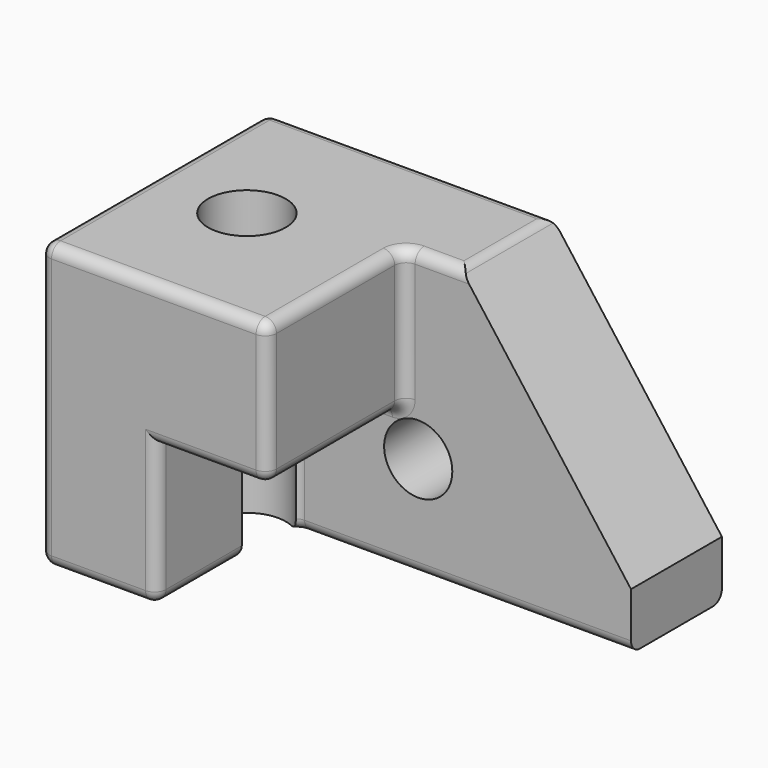
from build123d import *

# Parameters (mm, degrees)
F0_W     = 203.2
F0_H     = 127
F1_DEPTH = 127
F3_DEPTH = 76.2
F4_SIZE2 = 101.6
F4_SIZE  = 76.2
F5_R     = 5.08
F6_R     = 15.24
F7_DEPTH = 50.8
F8_R     = 17.3644725526
F9_DEPTH = 127


with BuildPart() as f1:
    # F0 (on Front) → F1 (new body)
    with BuildSketch(Plane.XZ):
        Rectangle(F0_W, F0_H)
    extrude(amount=F1_DEPTH)

    # F2 (on face) → F3 (cut)
    with BuildSketch(Plane.XZ.offset(127)):
        Polygon((101.6, 63.5), (0, 63.5), (0, 0), (-49.4145452976, 0), (-49.4145452976, -63.5), (101.6, -63.5), align=None)
    extrude(amount=-F3_DEPTH, mode=Mode.SUBTRACT)

    # F4
    f4_edges = [f1.edges().sort_by_distance(p)[0] for p in [
        (101.6, -25.4, 63.5),
    ]]
    f4_side = f1.faces().sort_by_distance((-21.771429, -52.614286, 63.5))[0]
    chamfer(f4_edges, length=F4_SIZE, length2=F4_SIZE2, reference=f4_side)

    # F5
    f5_edges = [f1.edges().sort_by_distance(p)[0] for p in [
        (25.4, -25.4, 63.5),
        (12.7, -50.8, 63.5),
        (0, -88.9, 63.5),
        (-50.8, -127, 63.5),
        (-101.6, -63.5, 63.5),
        (-38.1, 0, 63.5),
        (-101.6, -127, 0),
        (-49.414545, -127, -31.75),
        (-24.707273, -127, 0),
        (0, -88.9, 0),
        (0, -127, 31.75),
        (-75.507273, -127, -63.5),
        (0, -50.8, 31.75),
        (-101.6, 0, 0),
        (-101.6, -63.5, -63.5),
        (0, 0, -63.5),
        (26.092727, -50.8, -63.5),
        (-49.414545, -88.9, -63.5),
        (-49.414545, -50.8, -31.75),
        (-24.707273, -50.8, 0),
    ]]
    fillet(f5_edges, radius=F5_R)

    # F6 (on face) → F7 (cut, through all)
    with BuildSketch(Plane.XZ.offset(50.8)):
        with Locations((6.4654547024, -17.78)):
            Circle(F6_R)
    extrude(amount=-F7_DEPTH, mode=Mode.SUBTRACT)

    # F8 (on face) → F9 (cut, through all)
    with BuildSketch(Plane.XY.offset(63.5)):
        with Locations((-58.8048510253, -64.9624243379)):
            Circle(F8_R)
    extrude(amount=-F9_DEPTH, mode=Mode.SUBTRACT)


solid = f1.part
